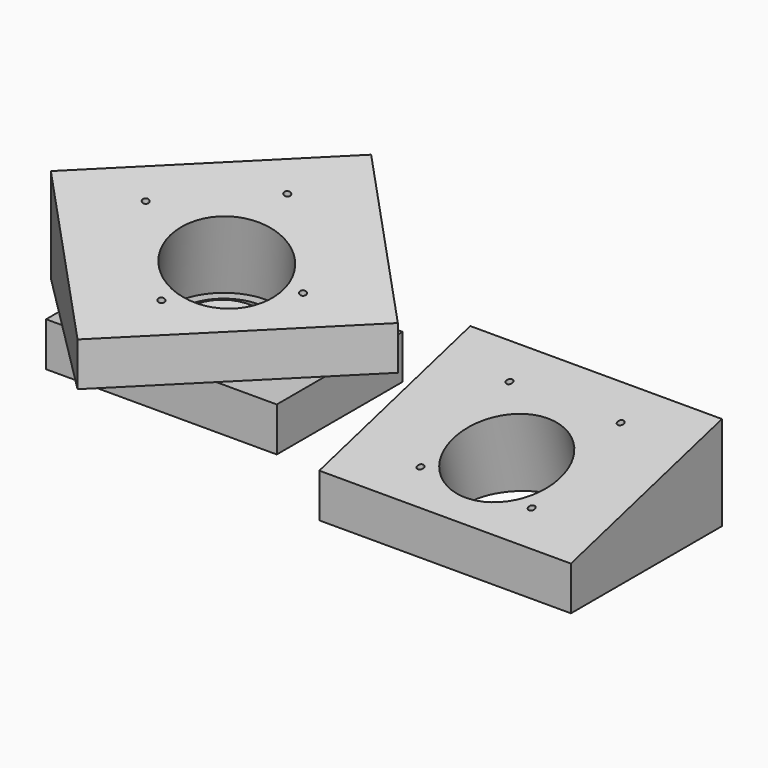
from build123d import *

# Parameters (mm, degrees)
F0_W      = 110
F0_H      = 75
F1_DEPTH  = 21
F3_DEPTH  = 45
F5_DEPTH  = 120
F6_R      = 25.5
F6_R_2    = 21
F7_DEPTH  = 40
F8_D      = 3
F9_DEPTH  = 38
F11_ANGLE = 45


# Not quite as in the source:
# - a feature names something its author has since deleted; it is built from what else it names


with BuildPart() as f1:
    # F0 (on Top) → F1 (new body)
    with BuildSketch(Plane.XY):
        Rectangle(F0_W, F0_H)
    extrude(amount=F1_DEPTH)

    # F6 (on face) → F9 (cut)
    with BuildSketch(Plane(origin=(9.535739116, -9.535739116, 50.3288383249), x_dir=(0.9831105487, 0.0340690567, -0.1798136492), z_dir=(0.1830127019, -0.1830127019, 0.9659258263))):
        with Locations((-3.7760866326, 3.9092925458)):
            Circle(F6_R_2)
    extrude(amount=-F9_DEPTH, mode=Mode.SUBTRACT)


with BuildPart() as f3:
    # F2 (on face) → F3 (new body)
    with BuildSketch(Plane.XY.offset(21)):
        Polygon((-74.2462120246, -10.6066017178), (-55, -29.8528137424), (-55, 8.6396103068), align=None)
        Polygon((26.1396103068, -37.5), (55, -8.6396103068), (55, 29.8528137424), (47.3528137424, 37.5), (-26.1396103068, 37.5), (-55, 8.6396103068), (-55, -29.8528137424), (-47.3528137424, -37.5), align=None)
        Polygon((-26.1396103068, 37.5), (47.3528137424, 37.5), (10.6066017178, 74.2462120246), align=None)
        Polygon((55, -8.6396103068), (74.2462120246, 10.6066017178), (55, 29.8528137424), align=None)
        Polygon((-10.6066017178, -74.2462120246), (26.1396103068, -37.5), (-47.3528137424, -37.5), align=None)
    extrude(amount=F3_DEPTH)

    # F4 (on face) → F5 (cut, through all)
    with BuildSketch(Plane(origin=(-42.4264068712, -42.4264068712, 0), x_dir=(0.7071067812, -0.7071067812, 0), z_dir=(-0.7071067812, -0.7071067812, 0))):
        Polygon((45, 66), (-45, 66), (45, 41.8845726812), align=None)
    extrude(amount=-F5_DEPTH, mode=Mode.SUBTRACT)

    # F6 (on face) → F7 (cut)
    with BuildSketch(Plane(origin=(9.535739116, -9.535739116, 50.3288383249), x_dir=(0.9831105487, 0.0340690567, -0.1798136492), z_dir=(0.1830127019, -0.1830127019, 0.9659258263))):
        with Locations((-3.7760866326, 3.9092925458)):
            Circle(F6_R)
        with Locations((-3.7760866326, 3.9092925458)):
            Circle(F6_R_2, mode=Mode.SUBTRACT)
        with Locations((-3.7760866326, 3.9092925458)):
            Circle(F6_R_2)
    extrude(amount=-F7_DEPTH, mode=Mode.SUBTRACT)

    # F8 (through all)
    with Locations(Plane(origin=(0, 0, 21), x_dir=(1, 0, 0), z_dir=(0, 0, -1))):
        with Locations((-37.5, 0), (0, 37.5), (37.5, 0), (0, -37.5)):
            Hole(F8_D / 2)


with BuildPart() as f10_1:
    # F10: copy of F3
    add(f3.part.moved(Location((200, 0, 0))))


with BuildPart() as f10_1_1:
    # F11: moved
    add(f10_1.part.rotate(Axis((125.7537879754, -10.6066017178, 43.5), (0, 0, -1)), F11_ANGLE))


solid = Compound([f1.part, f3.part, f10_1_1.part])
